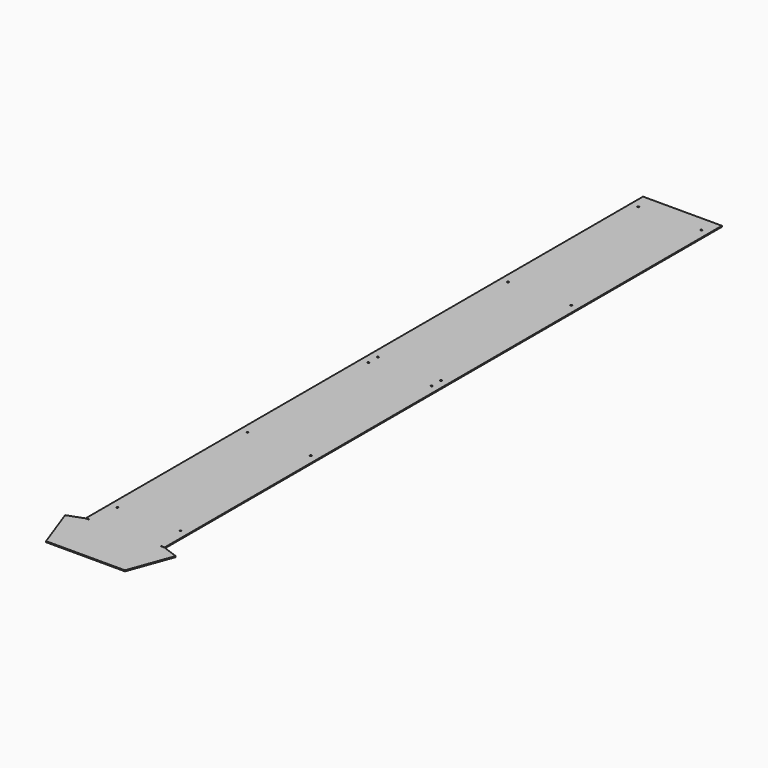
from build123d import *

# Parameters (mm, degrees)
F1_DEPTH = 5
F2_R     = 4.25
F3_DEPTH = 5.001
F4_R     = 4.25
F5_DEPTH = 5.001


# Not quite as in the source:
# - a pattern or mirror of a feature is missing from the dataset's text; its kind, count and spacing are read off the source's solid


with BuildPart() as f1:
    # F0 (on Top) → F1 (new body)
    with BuildSketch(Plane.XY):
        with BuildLine():
            Line((200, -1765), (200, 1765))
            Line((200, 1765), (-200, 1765))
            Line((-200, 1765), (-200, -1765))
            Line((-200, -1765), (-183, -1765))
            ThreePointArc((-183, -1765), (-182.6464466094, -1765.1464466094), (-182.5, -1765.5))
            Line((-182.5, -1765.5), (-182.5, -1766.5))
            ThreePointArc((-182.5, -1766.5), (-182.6464466094, -1766.8535533906), (-183, -1767))
            Line((-183, -1767), (-200, -1767))
            Line((-200, -1767), (-280.3484512108, -1796.2444446101))
            Line((-280.3484512108, -1796.2444446101), (-200, -2017))
            Line((-200, -2017), (200, -2017))
            Line((200, -2017), (280.3484512108, -1796.2444446101))
            Line((280.3484512108, -1796.2444446101), (200, -1767))
            Line((200, -1767), (183, -1767))
            ThreePointArc((183, -1767), (182.6464466094, -1766.8535533906), (182.5, -1766.5))
            Line((182.5, -1766.5), (182.5, -1765.5))
            ThreePointArc((182.5, -1765.5), (182.6464466094, -1765.1464466094), (183, -1765))
            Line((183, -1765), (200, -1765))
        make_face()
    extrude(amount=F1_DEPTH)

    # F2 (on face) → F3 (cut, through all)
    with BuildSketch(Plane.XY.offset(5)):
        with Locations((-160, 1685)):
            Circle(F2_R)
        with Locations((-160, 860)):
            Circle(F2_R)
        with Locations((-160, 35)):
            Circle(F2_R)
        with Locations((-160, -790)):
            Circle(F2_R)
        with Locations((-160, -1615)):
            Circle(F2_R)
    f3 = extrude(amount=-F3_DEPTH, mode=Mode.SUBTRACT)

    # F3_copies: F3 across plane
    add(f3.mirror(Plane(origin=(0, 0, 0), x_dir=(0, 0, 1), z_dir=(1, 0, 0))), mode=Mode.SUBTRACT)

    # F4 (on face) → F5 (cut, through all)
    with BuildSketch(Plane.XY.offset(5)):
        with Locations((-160, -25)):
            Circle(F4_R)
        with Locations((160, -25)):
            Circle(F4_R)
    extrude(amount=-F5_DEPTH, mode=Mode.SUBTRACT)


solid = f1.part
